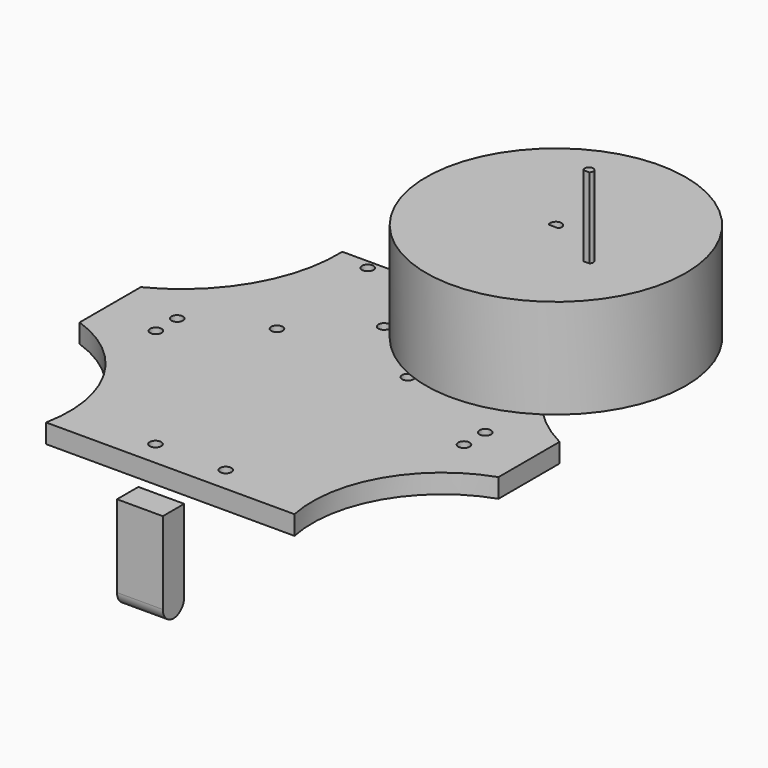
from build123d import *

# Parameters (mm, degrees)
F0_R      = 34
F1_DEPTH  = 26
F2_DEPTH  = 26
F3_W      = 10
F3_H      = 7
F4_DEPTH  = 22
F6_DEPTH  = 17
F7_R      = 1.5
F8_DEPTH  = 5
F9_W      = 12
F9_H      = 7
F10_DEPTH = 25
F11_R     = 3.49999
F12_DEPTH = 25
F14_DEPTH = 10


# Not quite as in the source:
# - a fillet or chamfer is up to 0.001 mm smaller than in the source, because OpenCascade refuses the exact size


with BuildPart() as f1:
    # F0 (on Top) → F1 (new body)
    with BuildSketch(Plane.XY):
        Circle(F0_R)
        with BuildLine():
            ThreePointArc((-1.2855, -0.7729746115), (0, 1.5), (1.2855, -0.7729746115))
            Line((1.2855, -0.7729746115), (-1.2855, -0.7729746115))
        make_face(mode=Mode.SUBTRACT)
    extrude(amount=F1_DEPTH)

    # F0 (on Top) → F2 (join)
    with BuildSketch(Plane.XY):
        Circle(F0_R)
        with BuildLine():
            ThreePointArc((-1.2855, -0.7729746115), (0, 1.5), (1.2855, -0.7729746115))
            Line((1.2855, -0.7729746115), (-1.2855, -0.7729746115))
        make_face(mode=Mode.SUBTRACT)
    extrude(amount=F2_DEPTH)


with BuildPart() as f4:
    # F3 (on Top) → F4 (new body)
    with BuildSketch(Plane.XY):
        with BuildLine():
            ThreePointArc((15.1895321906, -1.681498219), (12.2706510675, -2.4930327252), (10.1895321906, -4.6947137841))
            Line((10.1895321906, -4.6947137841), (20.1895321906, -4.6947137841))
            ThreePointArc((20.1895321906, -4.6947137841), (18.1084133136, -2.4930327252), (15.1895321906, -1.681498219))
        make_face()
        with BuildLine():
            Line((20.1895321906, -11.6947137841), (10.1895321906, -11.6947137841))
            ThreePointArc((10.1895321906, -11.6947137841), (12.2910870504, -13.8405250788), (15.1895321906, -14.6279606067))
            ThreePointArc((15.1895321906, -14.6279606067), (18.0879773307, -13.8405250788), (20.1895321906, -11.6947137841))
        make_face()
        with Locations((15.1895321906, -8.1947137841)):
            Rectangle(F3_W, F3_H)
    extrude(amount=F4_DEPTH)

    # F5 (on face) → F6 (join)
    with BuildSketch(Plane.XY.offset(22)):
        with BuildLine():
            Line((14.4120321906, -8.9939126017), (15.9670321906, -8.9939126017))
            ThreePointArc((15.9670321906, -8.9939126017), (15.1895321906, -7.0797137841), (14.4120321906, -8.9939126017))
        make_face()
    extrude(amount=F6_DEPTH)

    # F5 (on face) → F12 (join)
    with BuildSketch(Plane.XY.offset(22)):
        with BuildLine():
            Line((14.4120321906, -8.9939126017), (15.9670321906, -8.9939126017))
            ThreePointArc((15.9670321906, -8.9939126017), (15.1895321906, -7.0797137841), (14.4120321906, -8.9939126017))
        make_face()
    extrude(amount=F12_DEPTH)


with BuildPart() as f8:
    # F7 (on Top) → F8 (new body)
    with BuildSketch(Plane.XY):
        with BuildLine():
            Line((7.0208405241, 2.5), (-57.9437288691, 2.5))
            ThreePointArc((-57.9437288691, 2.5), (-63.5781988321, -19.7690987419), (-80.3373921663, -35.4786324501))
            Line((-80.3373921663, -35.4786324501), (-80.3373921663, -55.4786324501))
            ThreePointArc((-80.3373921663, -55.4786324501), (-61.8533257996, -70.7229983964), (-58.0151594759, -94.3729430437))
            Line((-58.0151594759, -94.3729430437), (-57.9791594759, -94.3729430437))
            Line((-57.9791594759, -94.3729430437), (7.0208405241, -94.3729430437))
            ThreePointArc((7.0208405241, -94.3729430437), (10.8617640259, -70.7277326236), (29.3427532497, -55.4862856296))
            Line((29.3427532497, -55.4862856296), (29.3427532497, -35.4862856296))
            ThreePointArc((29.3427532497, -35.4862856296), (12.6227799412, -19.7597925818), (7.0208405241, 2.5))
        make_face()
        with Locations((-34.5656405118, -87.8729430437)):
            Circle(F7_R, mode=Mode.SUBTRACT)
        with Locations((-65.8373921663, -48.6634840438)):
            Circle(F7_R, mode=Mode.SUBTRACT)
        with Locations((-16.1498492515, -87.8729430437)):
            Circle(F7_R, mode=Mode.SUBTRACT)
        with Locations((14.8427532497, -48.6634840438)):
            Circle(F7_R, mode=Mode.SUBTRACT)
        with Locations((-65.8373921663, -41.6857580474)):
            Circle(F7_R, mode=Mode.SUBTRACT)
        with Locations((-47.0499843359, -32.5)):
            Circle(F7_R, mode=Mode.SUBTRACT)
        with Locations((-30.5905751884, -18.0216301233)):
            Circle(F7_R, mode=Mode.SUBTRACT)
        with Locations((-49.4220566393, 0.1826457996)):
            Circle(F7_R, mode=Mode.SUBTRACT)
        with Locations((-12.7742653713, -32.5)):
            Circle(F7_R, mode=Mode.SUBTRACT)
        with Locations((14.8427532497, -41.6857580474)):
            Circle(F7_R, mode=Mode.SUBTRACT)
        with Locations((-1.5, 0)):
            Circle(F7_R, mode=Mode.SUBTRACT)
    extrude(amount=-F8_DEPTH)


with BuildPart() as f10:
    # F9 (on face) → F10 (new body)
    with BuildSketch(Plane(origin=(0, 0, -5), x_dir=(1, 0, 0), z_dir=(0, 0, -1))):
        with Locations((-25.4498492515, 100.8729430437)):
            Rectangle(F9_W, F9_H)
    extrude(amount=F10_DEPTH)

    # F11 (radius 3.5 in the source; OpenCascade refuses exactly that, so slightly less here)
    f11_edges = [f10.edges().sort_by_distance(p)[0] for p in [
        (-25.449849, -104.372943, -30),
        (-25.449849, -97.372943, -30),
    ]]
    fillet(f11_edges, radius=F11_R)


with BuildPart() as f14:
    # F13 (on Top) → F14 (new body)
    with BuildSketch(Plane.XY):
        with BuildLine():
            Line((-26.6139002144, 3.5212130751), (-34.6139002144, 3.5212130751))
            ThreePointArc((-34.6139002144, 3.5212130751), (-36.0281137768, 4.1069995128), (-36.6139002144, 5.5212130751))
            Line((-36.6139002144, 5.5212130751), (-36.6139002144, 8.5212130751))
            Line((-36.6139002144, 8.5212130751), (-37.5863661141, 8.5212130751))
            Line((-37.5863661141, 8.5212130751), (-37.5863661141, 2.867825795))
            Line((-37.5863661141, 2.867825795), (-23.7007507206, 2.867825795))
            Line((-23.7007507206, 2.867825795), (-23.7007507206, 8.5212130751))
            Line((-23.7007507206, 8.5212130751), (-24.6139002144, 8.5212130751))
            Line((-24.6139002144, 8.5212130751), (-24.6139002144, 5.5212130751))
            ThreePointArc((-24.6139002144, 5.5212130751), (-25.1996866521, 4.1069995128), (-26.6139002144, 3.5212130751))
        make_face()
    extrude(amount=F14_DEPTH)


solid = Compound([f1.part, f4.part, f8.part, f10.part, f14.part])
